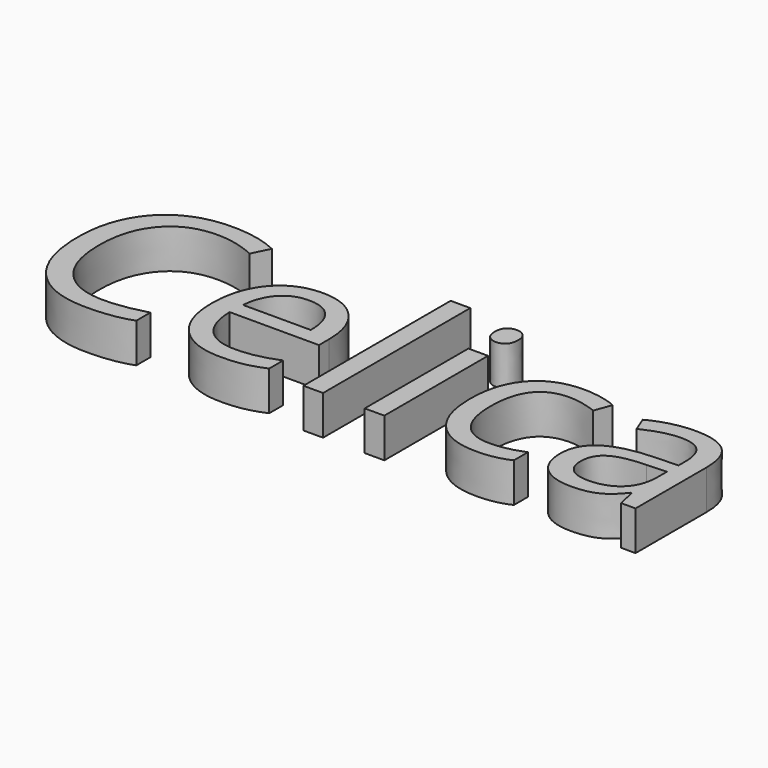
from build123d import *

# Parameters (mm, degrees)
F0_TEXT_SIZE = 39.0619135441
F1_DEPTH     = 6.35


# Not quite as in the source:
# - Text() gives the source's letters only with a copy of the font that has no kerning and outlines rounded to 1/6400 em; it was checked with that copy


with BuildPart() as f1:
    # F0 (on Top) → F1 (new body)
    with BuildSketch(Plane.XY):
        with Locations((-53.0082373642, 0)):
            Text('Celica', F0_TEXT_SIZE, font='Open Sans', text_align=(TextAlign.LEFT, TextAlign.BOTTOM))
    extrude(amount=F1_DEPTH)


solid = f1.part
